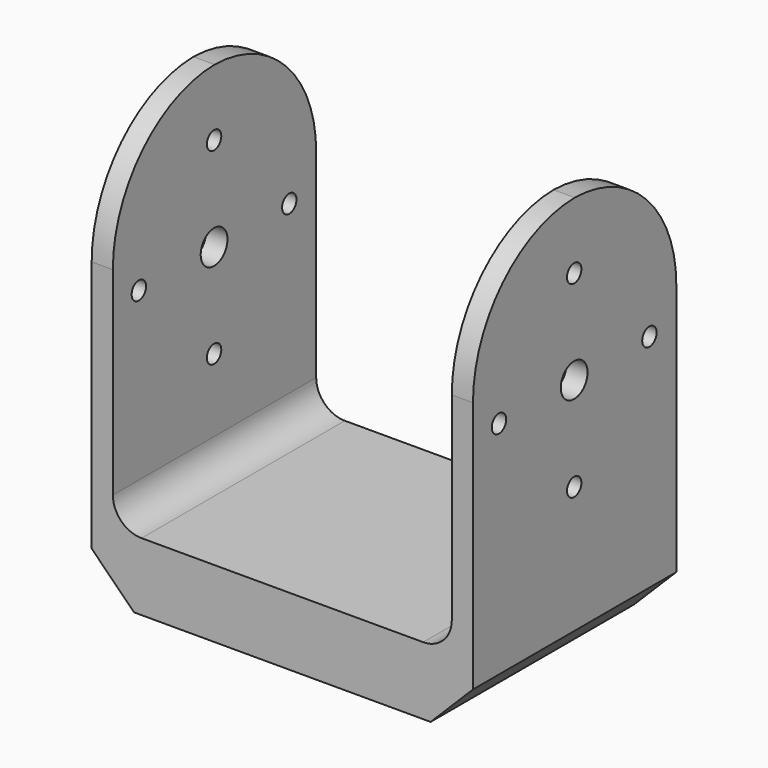
from build123d import *

# Parameters (mm, degrees)
F0_W        = 45
F0_H        = 50
F1_DEPTH    = 30
F2_W        = 40
F2_H        = 42
F3_DEPTH    = 30.001
F4_T1_DEPTH = 78.5477272148
F4_T3_DEPTH = 78.5477272148
F5_R        = 3.3798989873
F6_SIZE     = 5
F7_R        = 1.0624158
F7_R_2      = 1.974265
F8_DEPTH    = 45.001


# Not quite as in the source:
# - a fillet or chamfer that OpenCascade refuses, or shapes differently, is made with other operations: its cross-section is extruded or revolved along the edge and cut away or added


with BuildPart() as f1:
    # F0 (on Front) → F1 (new body)
    with BuildSketch(Plane.XZ):
        with Locations((5.6927716359, 6.5557161967)):
            Rectangle(F0_W, F0_H)
    extrude(amount=F1_DEPTH)

    # F2 (on face) → F3 (cut, through all)
    with BuildSketch(Plane.XZ.offset(30)):
        with Locations((5.6927716359, 10.5557161967)):
            Rectangle(F2_W, F2_H)
    extrude(amount=-F3_DEPTH, mode=Mode.SUBTRACT)

    # F4: fillet of radius 15.209545443 on 4 edges, made by hand

    # F4_s2 → F4_t1 (cut)
    with BuildSketch(Plane.YZ.offset(-54.8310919714)):
        with BuildLine():
            ThreePointArc((0, 16.3461707538), (-4.4547727215, 27.1009434752), (-15.209545443, 31.5557161967))
            Line((-15.209545443, 31.5557161967), (0, 31.5557161967))
            Line((0, 31.5557161967), (0, 16.3461707538))
        make_face()
        with BuildLine():
            ThreePointArc((-30, 16.3461707538), (-25.5452272785, 27.1009434752), (-14.790454557, 31.5557161967))
            Line((-14.790454557, 31.5557161967), (-30, 31.5557161967))
            Line((-30, 31.5557161967), (-30, 16.3461707538))
        make_face()
    extrude(amount=F4_T1_DEPTH, mode=Mode.SUBTRACT)

    # F4_s4 → F4_t3 (cut)
    with BuildSketch(Plane.YZ.offset(-12.3310919714)):
        with BuildLine():
            ThreePointArc((-14.790454557, 31.5557161967), (-25.5452272785, 27.1009434752), (-30, 16.3461707538))
            Line((-30, 16.3461707538), (-30, 31.5557161967))
            Line((-30, 31.5557161967), (-14.790454557, 31.5557161967))
        make_face()
        with BuildLine():
            ThreePointArc((-15.209545443, 31.5557161967), (-4.4547727215, 27.1009434752), (0, 16.3461707538))
            Line((0, 16.3461707538), (0, 31.5557161967))
            Line((0, 31.5557161967), (-15.209545443, 31.5557161967))
        make_face()
    extrude(amount=F4_T3_DEPTH, mode=Mode.SUBTRACT)

    # F5
    f5_edges = [f1.edges().sort_by_distance(p)[0] for p in [
        (-14.307228, -15, -10.444284),
        (25.692772, -15, -10.444284),
    ]]
    fillet(f5_edges, radius=F5_R)

    # F6
    f6_edges = [f1.edges().sort_by_distance(p)[0] for p in [
        (-16.807228, -15, -18.444284),
        (28.192772, -15, -18.444284),
    ]]
    chamfer(f6_edges, length=F6_SIZE)

    # F7 (on face) → F8 (cut, through all)
    with BuildSketch(Plane(origin=(-16.8072283641, 0, 0), x_dir=(0, -1, 0), z_dir=(-1, 0, 0))):
        with Locations((3.9704506522, 12.6322340244)):
            Circle(F7_R)
        with Locations((15.0680806522, 23.7298640244)):
            Circle(F7_R)
        with Locations((26.1657106522, 12.6322340244)):
            Circle(F7_R)
        with Locations((15.0680806522, 1.5346040244)):
            Circle(F7_R)
        with Locations((15.0680806522, 12.6322340244)):
            Circle(F7_R_2)
    extrude(amount=-F8_DEPTH, mode=Mode.SUBTRACT)


solid = f1.part
